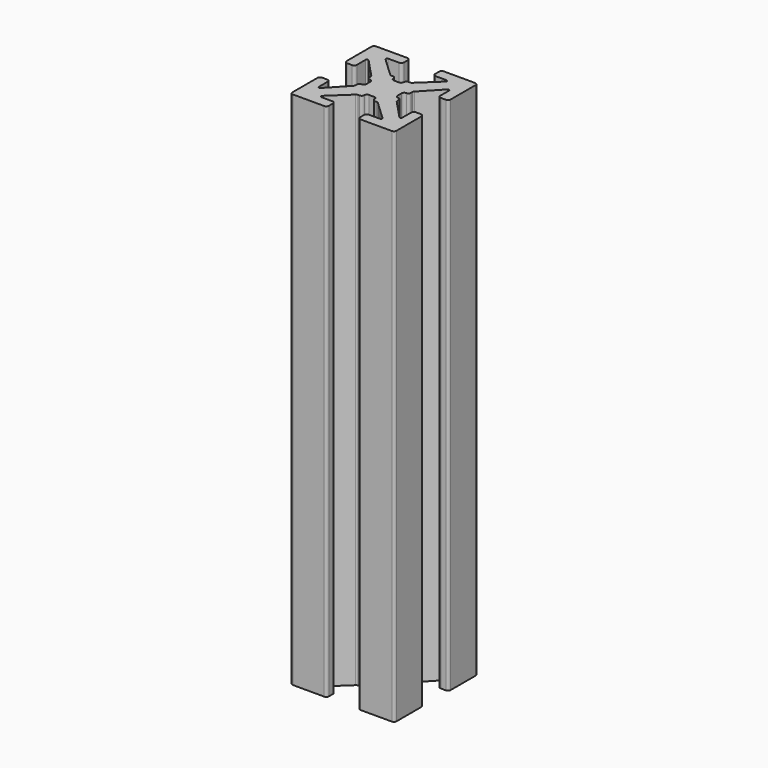
from build123d import *

# Parameters (mm, degrees)
F1_DEPTH = 25


# Not quite as in the source:
# - ends of sketch curves that miss each other by under 0.0002 mm in the source are joined


with BuildPart() as f1:
    # F0 (on Top) → F1 (new body, symmetric)
    with BuildSketch(Plane.XY):
        with BuildLine():
            ThreePointArc((2.803779, 4.0132), (2.9218403787, 3.9330028938), (2.8907965459, 3.7936962341))
            Line((2.8907965459, 3.7936962341), (1.0639298, 2.075561))
            ThreePointArc((1.0639298, 2.075561), (0.9835034993, 2.0244706276), (0.8899144, 2.0066))
            Line((0.8899144, 2.0066), (0.7493, 2.0066))
            ThreePointArc((0.7493, 2.0066), (0.5696948776, 1.9322051224), (0.4953, 1.7526))
            ThreePointArc((0.4953, 1.7526), (0.4209051224, 1.5729948776), (0.2413, 1.4986))
            Line((0.2413, 1.4986), (-0.2413, 1.4986))
            ThreePointArc((-0.2413, 1.4986), (-0.4209051224, 1.5729948776), (-0.4953, 1.7526))
            ThreePointArc((-0.4953, 1.7526), (-0.5696948776, 1.9322051224), (-0.7493, 2.0066))
            Line((-0.7493, 2.0066), (-0.8899144, 2.0066))
            ThreePointArc((-0.8899144, 2.0066), (-0.9835034993, 2.0244706276), (-1.0639233392, 2.0755678701))
            Line((-1.0639233392, 2.0755678701), (-2.8907994, 3.7936932))
            ThreePointArc((-2.8907994, 3.7936932), (-2.9218403787, 3.9330028938), (-2.803779, 4.0132))
            Line((-2.803779, 4.0132), (-1.7526, 4.0132))
            ThreePointArc((-1.7526, 4.0132), (-1.5729948776, 4.0875948776), (-1.4986, 4.2672))
            Line((-1.4986, 4.2672), (-1.4986, 4.7498))
            ThreePointArc((-1.4986, 4.7498), (-1.5729948776, 4.9294051224), (-1.7526, 5.0038))
            Line((-1.7526, 5.0038), (-4.7498, 5.0038))
            ThreePointArc((-4.7498, 5.0038), (-4.9294051224, 4.9294051224), (-5.0038, 4.7498))
            Line((-5.0038, 4.7498), (-5.0038, 1.7526))
            ThreePointArc((-5.0038, 1.7526), (-4.9294051224, 1.5729948776), (-4.7498, 1.4986))
            Line((-4.7498, 1.4986), (-4.2672, 1.4986))
            ThreePointArc((-4.2672, 1.4986), (-4.0875948776, 1.5729948776), (-4.0132, 1.7526))
            Line((-4.0132, 1.7526), (-4.0132, 2.803779))
            ThreePointArc((-4.0132, 2.803779), (-3.9330028938, 2.9218403787), (-3.7936962341, 2.8907965459))
            Line((-3.7936962341, 2.8907965459), (-2.075561, 1.0639298))
            ThreePointArc((-2.075561, 1.0639298), (-2.0244706276, 0.9835034993), (-2.0066, 0.8899144))
            Line((-2.0066, 0.8899144), (-2.0066, 0.7493))
            ThreePointArc((-2.0066, 0.7493), (-1.9322051224, 0.5696948776), (-1.7526, 0.4953))
            ThreePointArc((-1.7526, 0.4953), (-1.5729948776, 0.4209051224), (-1.4986, 0.2413))
            Line((-1.4986, 0.2413), (-1.4986, -0.2413))
            ThreePointArc((-1.4986, -0.2413), (-1.5729948776, -0.4209051224), (-1.7526, -0.4953))
            ThreePointArc((-1.7526, -0.4953), (-1.9322051224, -0.5696948776), (-2.0066, -0.7493))
            Line((-2.0066, -0.7493), (-2.0066, -0.8899144))
            ThreePointArc((-2.0066, -0.8899144), (-2.0244706276, -0.9835034993), (-2.0755678701, -1.0639233392))
            Line((-2.0755678701, -1.0639233392), (-3.7936932, -2.8907994))
            ThreePointArc((-3.7936932, -2.8907994), (-3.9330028938, -2.9218403787), (-4.0132, -2.803779))
            Line((-4.0132, -2.803779), (-4.0132, -1.7526))
            ThreePointArc((-4.0132, -1.7526), (-4.0875948776, -1.5729948776), (-4.2672, -1.4986))
            Line((-4.2672, -1.4986), (-4.7498, -1.4986))
            ThreePointArc((-4.7498, -1.4986), (-4.9294051224, -1.5729948776), (-5.0038, -1.7526))
            Line((-5.0038, -1.7526), (-5.0038, -4.7498))
            ThreePointArc((-5.0038, -4.7498), (-4.9294051224, -4.9294051224), (-4.7498, -5.0038))
            Line((-4.7498, -5.0038), (-1.7526, -5.0038))
            ThreePointArc((-1.7526, -5.0038), (-1.5729948776, -4.9294051224), (-1.4986, -4.7498))
            Line((-1.4986, -4.7498), (-1.4986, -4.2672))
            ThreePointArc((-1.4986, -4.2672), (-1.5729948776, -4.0875948776), (-1.7526, -4.0132))
            Line((-1.7526, -4.0132), (-2.803779, -4.0132))
            ThreePointArc((-2.803779, -4.0132), (-2.9218403787, -3.9330028938), (-2.8907965459, -3.7936962341))
            Line((-2.8907965459, -3.7936962341), (-1.0639298, -2.075561))
            ThreePointArc((-1.0639298, -2.075561), (-0.9835034993, -2.0244706276), (-0.8899144, -2.0066))
            Line((-0.8899144, -2.0066), (-0.7493, -2.0066))
            ThreePointArc((-0.7493, -2.0066), (-0.5696948776, -1.9322051224), (-0.4953, -1.7526))
            ThreePointArc((-0.4953, -1.7526), (-0.4209051224, -1.5729948776), (-0.2413, -1.4986))
            Line((-0.2413, -1.4986), (0.2413, -1.4986))
            ThreePointArc((0.2413, -1.4986), (0.4209051224, -1.5729948776), (0.4953, -1.7526))
            ThreePointArc((0.4953, -1.7526), (0.5696948776, -1.9322051224), (0.7493, -2.0066))
            Line((0.7493, -2.0066), (0.8899144, -2.0066))
            ThreePointArc((0.8899144, -2.0066), (0.9835034993, -2.0244706276), (1.0639233392, -2.0755678701))
            Line((1.0639233392, -2.0755678701), (2.8907994, -3.7936932))
            ThreePointArc((2.8907994, -3.7936932), (2.9218403787, -3.9330028938), (2.803779, -4.0132))
            Line((2.803779, -4.0132), (1.7526, -4.0132))
            ThreePointArc((1.7526, -4.0132), (1.5729948776, -4.0875948776), (1.4986, -4.2672))
            Line((1.4986, -4.2672), (1.4986, -4.7498))
            ThreePointArc((1.4986, -4.7498), (1.5729948776, -4.9294051224), (1.7526, -5.0038))
            Line((1.7526, -5.0038), (4.7498, -5.0038))
            ThreePointArc((4.7498, -5.0038), (4.9294051224, -4.9294051224), (5.0038, -4.7498))
            Line((5.0038, -4.7498), (5.0038, -1.7526))
            ThreePointArc((5.0038, -1.7526), (4.9294051224, -1.5729948776), (4.7498, -1.4986))
            Line((4.7498, -1.4986), (4.2672, -1.4986))
            ThreePointArc((4.2672, -1.4986), (4.0875948776, -1.5729948776), (4.0132, -1.7526))
            Line((4.0132, -1.7526), (4.0132, -2.803779))
            ThreePointArc((4.0132, -2.803779), (3.9330028938, -2.9218403787), (3.7936962341, -2.8907965459))
            Line((3.7936962341, -2.8907965459), (2.075561, -1.0639298))
            ThreePointArc((2.075561, -1.0639298), (2.0244706276, -0.9835034993), (2.0066, -0.8899144))
            Line((2.0066, -0.8899144), (2.0066, -0.7493))
            ThreePointArc((2.0066, -0.7493), (1.9322051224, -0.5696948776), (1.7526, -0.4953))
            ThreePointArc((1.7526, -0.4953), (1.5729948776, -0.4209051224), (1.4986, -0.2413))
            Line((1.4986, -0.2413), (1.4986, 0.2413))
            ThreePointArc((1.4986, 0.2413), (1.5729948776, 0.4209051224), (1.7526, 0.4953))
            ThreePointArc((1.7526, 0.4953), (1.9322051224, 0.5696948776), (2.0066, 0.7493))
            Line((2.0066, 0.7493), (2.0066, 0.8899144))
            ThreePointArc((2.0066, 0.8899144), (2.0244706276, 0.9835034993), (2.0755678701, 1.0639233392))
            Line((2.0755678701, 1.0639233392), (3.7936932, 2.8907994))
            ThreePointArc((3.7936932, 2.8907994), (3.9330028938, 2.9218403787), (4.0132, 2.803779))
            Line((4.0132, 2.803779), (4.0132, 1.7526))
            ThreePointArc((4.0132, 1.7526), (4.0875948776, 1.5729948776), (4.2672, 1.4986))
            Line((4.2672, 1.4986), (4.7498, 1.4986))
            ThreePointArc((4.7498, 1.4986), (4.9294051224, 1.5729948776), (5.0038, 1.7526))
            Line((5.0038, 1.7526), (5.0038, 4.7498))
            ThreePointArc((5.0038, 4.7498), (4.9294051224, 4.9294051224), (4.7498, 5.0038))
            Line((4.7498, 5.0038), (1.7526, 5.0038))
            ThreePointArc((1.7526, 5.0038), (1.5729948776, 4.9294051224), (1.4986, 4.7498))
            Line((1.4986, 4.7498), (1.4986, 4.2672))
            ThreePointArc((1.4986, 4.2672), (1.5729948776, 4.0875948776), (1.7526, 4.0132))
            Line((1.7526, 4.0132), (2.803779, 4.0132))
        make_face()
    extrude(amount=F1_DEPTH, both=True)


solid = f1.part
